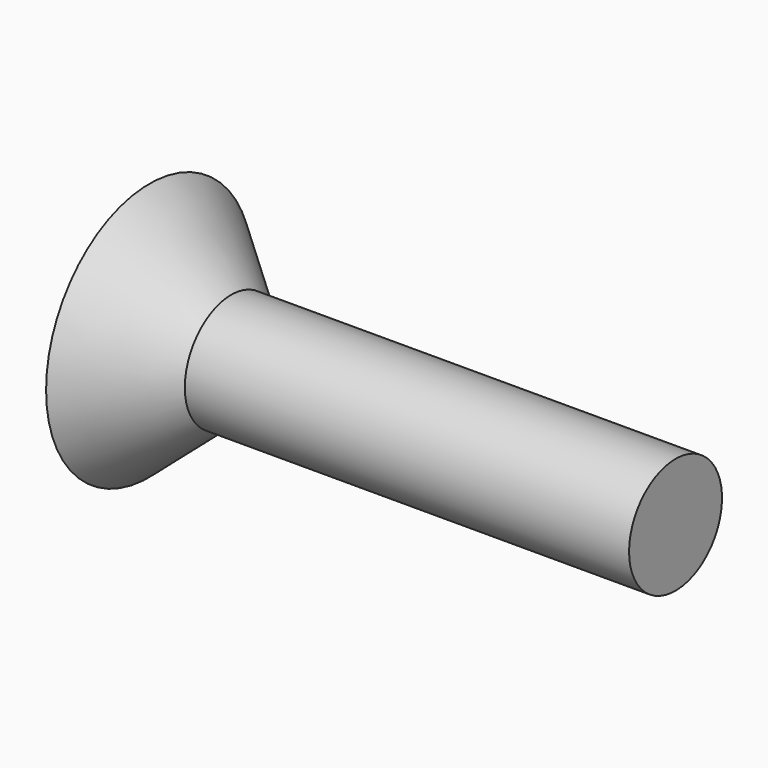
from build123d import *

# Parameters (mm, degrees)
F4_DEPTH = 2.286


# Not quite as in the source:
# - a feature names something its author has since deleted; it is built from what else it names


with BuildPart() as f2:
    # F0 (on Top) → F2 (revolve)
    with BuildSketch(Plane.XY):
        Polygon((2.4690357124, -1.7526), (15.875, -1.7526), (15.875, 0), (0, 0), (0, -3.8989), align=None)
    revolve(axis=Axis((4.9627271947, 0, 0), (1, 0, 0)))

    # F3 (on face) → F4 (cut)
    with BuildSketch(Plane(origin=(0, 0, 0), x_dir=(0, -1, 0), z_dir=(-1, 0, 0))):
        Polygon((0.5728397202, 0.9921875), (-0.5728397202, 0.9921875), (-1.1456794404, 0), (-0.5728397202, -0.9921875), (0.5728397202, -0.9921875), (1.1456794404, 0), align=None)
    extrude(amount=-F4_DEPTH, mode=Mode.SUBTRACT)


solid = f2.part
